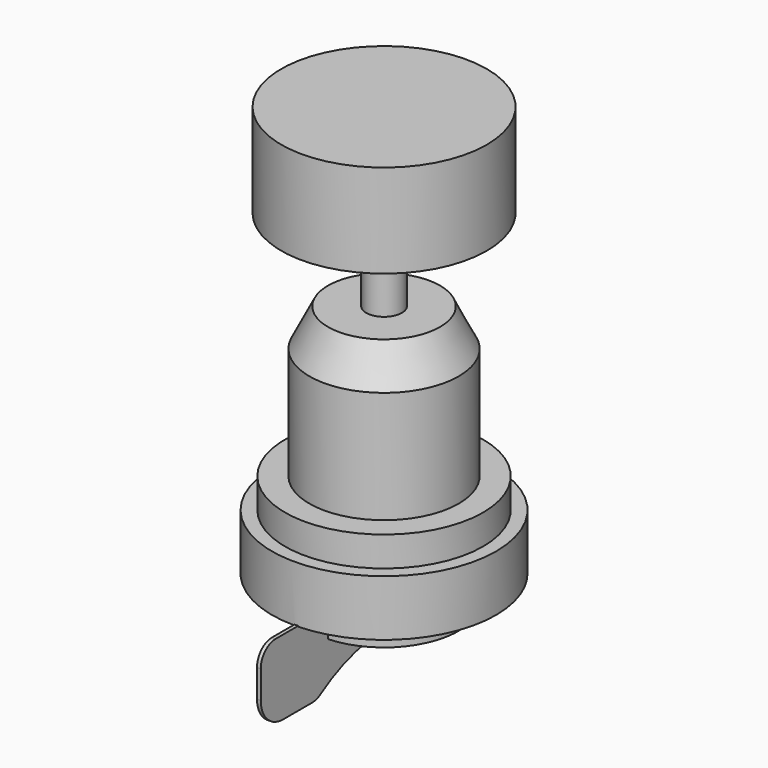
from build123d import *

# Parameters (mm, degrees)
F0_R      = 30
F1_DEPTH  = 15
F2_R      = 26.5
F3_DEPTH  = 8
F4_R      = 20
F5_DEPTH  = 40
F6_R      = 20
F7_DEPTH  = 7
F9_DEPTH  = 1
F11_DEPTH = 25
F12_R     = 5
F13_SIZE2 = 10
F13_SIZE  = 5
F14_R     = 1
F15_DEPTH = 15
F16_R     = 4.7918026285
F16_R_2   = 1
F17_DEPTH = 22
F18_R     = 27.5
F18_R_2   = 4.7918026285
F19_DEPTH = 25


# Not quite as in the source:
# - a feature names something its author has since deleted; it is built from what else it names


with BuildPart() as f1:
    # F0 (on Top) → F1 (new body)
    with BuildSketch(Plane.XY):
        Circle(F0_R)
    extrude(amount=F1_DEPTH)

    # F2 (on face) → F3 (join)
    with BuildSketch(Plane.XY.offset(15)):
        Circle(F2_R)
    extrude(amount=F3_DEPTH)

    # F4 (on face) → F5 (join)
    with BuildSketch(Plane.XY.offset(23)):
        Circle(F4_R)
    extrude(amount=F5_DEPTH)

    # F6 (on face) → F7 (join)
    with BuildSketch(Plane(origin=(0, 0, 0), x_dir=(1, 0, 0), z_dir=(0, 0, -1))):
        Circle(F6_R)
    extrude(amount=F7_DEPTH)

    # F8 (on Right) → F9 (join)
    with BuildSketch(Plane.YZ):
        with BuildLine():
            Line((37.5, 0.200964841), (0, 0.200964841))
            Line((0, 0.200964841), (0, -19.799035159))
            Line((0, -19.799035159), (35, -19.799035159))
            ThreePointArc((35, -19.799035159), (40.3033008589, -17.6023360179), (42.5, -12.299035159))
            Line((42.5, -12.299035159), (42.5, -4.799035159))
            ThreePointArc((42.5, -4.799035159), (41.0355339059, -1.2635012531), (37.5, 0.200964841))
        make_face()
        with BuildLine():
            Line((0, -19.799035159), (0, 0.200964841))
            Line((0, 0.200964841), (-37.5, 0.200964841))
            ThreePointArc((-37.5, 0.200964841), (-41.0355339059, -1.2635012531), (-42.5, -4.799035159))
            Line((-42.5, -4.799035159), (-42.5, -12.299035159))
            ThreePointArc((-42.5, -12.299035159), (-40.3033008589, -17.6023360179), (-35, -19.799035159))
            Line((-35, -19.799035159), (0, -19.799035159))
        make_face()
    extrude(amount=F9_DEPTH)

    # F10 (on face) → F11 (cut)
    with BuildSketch(Plane.YZ.offset(1)):
        with BuildLine():
            Line((-23.7842038121, -19.799035159), (23.7842038121, -19.799035159))
            ThreePointArc((23.7842038121, -19.799035159), (0, -12.2829212631), (-23.7842038121, -19.799035159))
        make_face()
    extrude(amount=-F11_DEPTH, mode=Mode.SUBTRACT)

    # F12
    f12_edges = [f1.edges().sort_by_distance(p)[0] for p in [
        (0.5, -23.784204, -19.799035),
        (0.5, 23.784204, -19.799035),
    ]]
    fillet(f12_edges, radius=F12_R)

    # F13
    f13_edges = [f1.edges().sort_by_distance(p)[0] for p in [
        (-20, 0, 63),
    ]]
    f13_side = f1.faces().sort_by_distance((0, 0, 63))[0]
    chamfer(f13_edges, length=F13_SIZE, length2=F13_SIZE2, reference=f13_side)

    # F14 (on face) → F15 (join)
    with BuildSketch(Plane.XY.offset(63)):
        Circle(F14_R)
    extrude(amount=F15_DEPTH)

    # F16 (on face) → F17 (join)
    with BuildSketch(Plane.XY.offset(63)):
        Circle(F16_R)
        Circle(F16_R_2, mode=Mode.SUBTRACT)
        Circle(F16_R_2)
    extrude(amount=F17_DEPTH)

    # F18 (on face) → F19 (join)
    with BuildSketch(Plane.XY.offset(85)):
        Circle(F18_R)
        Circle(F18_R_2, mode=Mode.SUBTRACT)
        Circle(F18_R_2)
    extrude(amount=F19_DEPTH)


solid = f1.part
